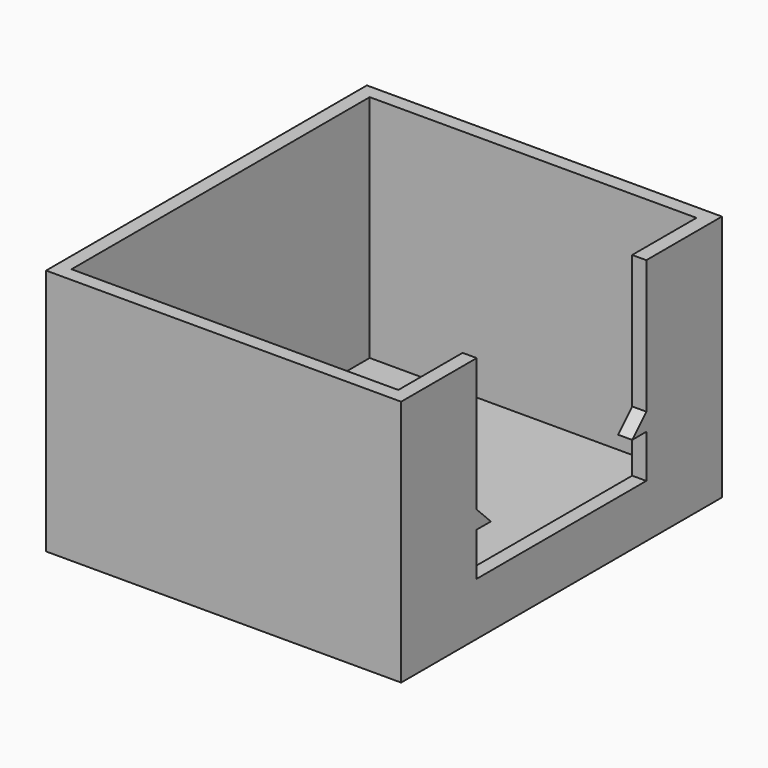
from build123d import *

# Parameters (mm, degrees)
F0_W        = 20.1
F0_H        = 22.7
F0_W_2      = 18.5
F0_H_2      = 21.1
F1_DEPTH    = 14
F2_DEPTH    = 1
F3_W        = 0.8
F3_H        = 12
F4_DEPTH    = 11
F5_W        = 0.8
F5_H        = 2
F6_DEPTH    = 1
F7_W        = 0.8
F7_H        = 2
F8_DEPTH    = 1
F9_T4_DEPTH = 11.0867319519
F9_T9_DEPTH = 11.0867319519


# Not quite as in the source:
# - a fillet or chamfer that OpenCascade refuses, or shapes differently, is made with other operations: its cross-section is extruded or revolved along the edge and cut away or added


with BuildPart() as f1:
    # F0 (on Top) → F1 (new body)
    with BuildSketch(Plane.XY):
        Rectangle(F0_W, F0_H)
        Rectangle(F0_W_2, F0_H_2, mode=Mode.SUBTRACT)
    extrude(amount=F1_DEPTH)

    # F0 (on Top) → F2 (join)
    with BuildSketch(Plane.XY):
        Rectangle(F0_W_2, F0_H_2)
    extrude(amount=F2_DEPTH)

    # F3 (on face) → F4 (cut)
    with BuildSketch(Plane.XY.offset(14)):
        with Locations((9.65, 0)):
            Rectangle(F3_W, F3_H)
    extrude(amount=-F4_DEPTH, mode=Mode.SUBTRACT)

    # F5 (on face) → F6 (join)
    with BuildSketch(Plane.XZ.offset(-6)):
        with Locations((9.65, 6.45)):
            Rectangle(F5_W, F5_H)
    extrude(amount=F6_DEPTH)

    # F7 (on face) → F8 (join)
    with BuildSketch(Plane(origin=(0, -6, 0), x_dir=(-1, 0, 0), z_dir=(0, 1, 0))):
        with Locations((-9.65, 6.45)):
            Rectangle(F7_W, F7_H)
    extrude(amount=F8_DEPTH)

    # F9: chamfer of 2 on 2 edges, made by hand


with BuildPart() as f9_tool2:
    # F9_s3 → F9_t4 (new body)
    with BuildSketch(Plane.YZ.offset(15.1933659759)):
        Polygon((5, 5.45), (7, 7.45), (5, 7.45), align=None)
    extrude(amount=-F9_T4_DEPTH)

    split(bisect_by=Plane.XZ.offset(-6), keep=Keep.TOP)


with BuildPart() as f1_1:
    add(f1.part)

    # F9_t1: cut F9_tool2
    add(f9_tool2.part, mode=Mode.SUBTRACT)


with BuildPart() as f9_tool7:
    # F9_s8 → F9_t9 (new body)
    with BuildSketch(Plane.YZ.offset(4.1066340241)):
        Polygon((-7, 7.45), (-5, 5.45), (-5, 7.45), align=None)
    extrude(amount=F9_T9_DEPTH)

    split(bisect_by=Plane.XZ.offset(6), keep=Keep.BOTTOM)


with BuildPart() as f1_2:
    add(f1_1.part)

    # F9_t6: cut F9_tool7
    add(f9_tool7.part, mode=Mode.SUBTRACT)


solid = f1_2.part
